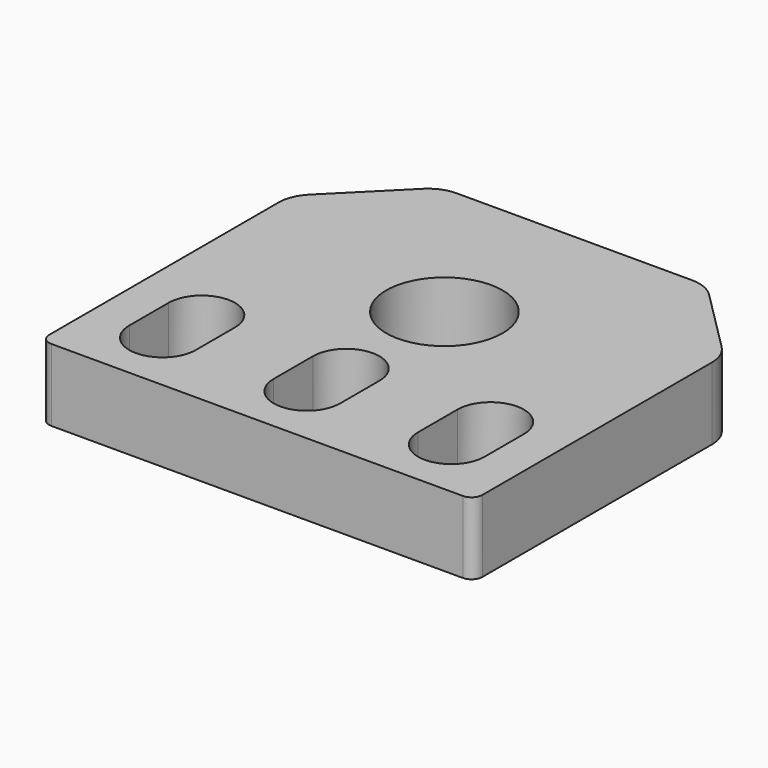
from build123d import *

# Parameters (mm, degrees)
F0_R     = 8.05
F1_DEPTH = 10
F2_DEPTH = 3


# Not quite as in the source:
# - ends of sketch curves that miss each other by under 0.0002 mm in the source are joined


with BuildPart() as f1:
    # F0 (on Top) → F1 (new body)
    with BuildSketch(Plane.XY):
        with BuildLine():
            ThreePointArc((-16.278933, 27.465), (-18.1923501618, 27.0843976626), (-19.8144669059, 26.0005339059))
            Line((-19.8144669059, 26.0005339059), (-28.535534, 17.279466))
            ThreePointArc((-28.535534, 17.279466), (-29.6193976626, 15.6573491618), (-30, 13.743932))
            Line((-30, 13.743932), (-30, -25.965))
            ThreePointArc((-30, -25.965), (-29.5606601718, -27.0256601718), (-28.5, -27.465))
            Line((-28.5, -27.465), (28.5, -27.465))
            ThreePointArc((28.5, -27.465), (29.5606601718, -27.0256601718), (30, -25.965))
            Line((30, -25.965), (30, 13.743932))
            ThreePointArc((30, 13.743932), (29.6193976626, 15.6573491618), (28.5355339059, 17.2794659059))
            Line((28.5355339059, 17.2794659059), (19.814466, 26.000533))
            ThreePointArc((19.814466, 26.000533), (18.1923494885, 27.0843975273), (16.278932, 27.465))
            Line((16.278932, 27.465), (-16.278933, 27.465))
        make_face()
        with BuildLine():
            ThreePointArc((-24.6, -12.035), (-20, -7.435), (-15.4, -12.035))
            Line((-15.4, -12.035), (-15.4, -18.835))
            ThreePointArc((-15.4, -18.835), (-20, -23.435), (-24.6, -18.835))
            Line((-24.6, -18.835), (-24.6, -12.035))
        make_face(mode=Mode.SUBTRACT)
        with BuildLine():
            ThreePointArc((4.6, -18.835), (0, -23.435), (-4.6, -18.835))
            Line((-4.6, -18.835), (-4.6, -12.035))
            ThreePointArc((-4.6, -12.035), (0, -7.435), (4.6, -12.035))
            Line((4.6, -12.035), (4.6, -18.835))
        make_face(mode=Mode.SUBTRACT)
        with BuildLine():
            ThreePointArc((15.4, -12.035), (20, -7.435), (24.6, -12.035))
            Line((24.6, -12.035), (24.6, -18.835))
            ThreePointArc((24.6, -18.835), (20, -23.435), (15.4, -18.835))
            Line((15.4, -18.835), (15.4, -12.035))
        make_face(mode=Mode.SUBTRACT)
        with Locations((0, 4.965)):
            Circle(F0_R, mode=Mode.SUBTRACT)
    extrude(amount=F1_DEPTH)

    # F0 (on Top) → F2 (join)
    with BuildSketch(Plane.XY):
        with BuildLine():
            Line((-15.4, -18.835), (-15.4, -12.035))
            ThreePointArc((-15.4, -12.035), (-20, -7.435), (-24.6, -12.035))
            Line((-24.6, -12.035), (-24.6, -18.835))
            ThreePointArc((-24.6, -18.835), (-20, -23.435), (-15.4, -18.835))
        make_face()
        with BuildLine():
            ThreePointArc((-17.5, -18.835), (-20, -21.335), (-22.5, -18.835))
            Line((-22.5, -18.835), (-22.5, -12.035))
            ThreePointArc((-22.5, -12.035), (-20, -9.535), (-17.5, -12.035))
            Line((-17.5, -12.035), (-17.5, -18.835))
        make_face(mode=Mode.SUBTRACT)
        with BuildLine():
            Line((-4.6, -12.035), (-4.6, -18.835))
            ThreePointArc((-4.6, -18.835), (0, -23.435), (4.6, -18.835))
            Line((4.6, -18.835), (4.6, -12.035))
            ThreePointArc((4.6, -12.035), (0, -7.435), (-4.6, -12.035))
        make_face()
        with BuildLine():
            ThreePointArc((2.5, -18.835), (0, -21.335), (-2.5, -18.835))
            Line((-2.5, -18.835), (-2.5, -12.035))
            ThreePointArc((-2.5, -12.035), (0, -9.535), (2.5, -12.035))
            Line((2.5, -12.035), (2.5, -18.835))
        make_face(mode=Mode.SUBTRACT)
        with BuildLine():
            Line((24.6, -18.835), (24.6, -12.035))
            ThreePointArc((24.6, -12.035), (20, -7.435), (15.4, -12.035))
            Line((15.4, -12.035), (15.4, -18.835))
            ThreePointArc((15.4, -18.835), (20, -23.435), (24.6, -18.835))
        make_face()
        with BuildLine():
            ThreePointArc((22.5, -18.835), (20, -21.335), (17.5, -18.835))
            Line((17.5, -18.835), (17.5, -12.035))
            ThreePointArc((17.5, -12.035), (20, -9.535), (22.5, -12.035))
            Line((22.5, -12.035), (22.5, -18.835))
        make_face(mode=Mode.SUBTRACT)
    extrude(amount=F2_DEPTH)


solid = f1.part
